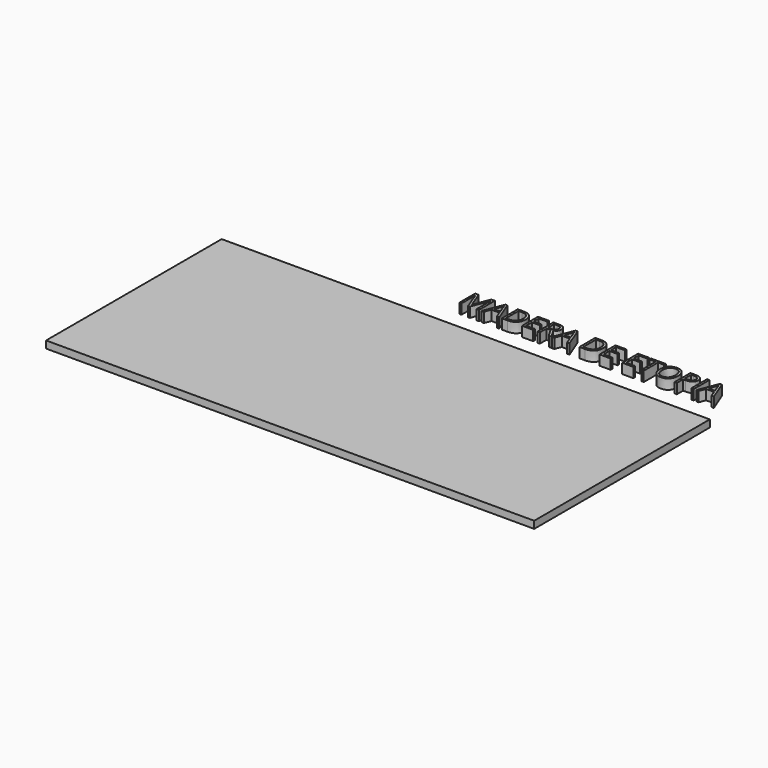
from build123d import *

# Parameters (mm, degrees)
F0_W         = 1223
F0_H         = 550
F1_DEPTH     = 18
F2_TEXT_SIZE = 69.4444444444
F3_DEPTH     = 25


# Not quite as in the source:
# - Text() gives the source's letters only with a copy of the font that has no kerning and outlines rounded to 1/6400 em; it was checked with that copy


with BuildPart() as f1:
    # F0 (on Top) → F1 (new body)
    with BuildSketch(Plane.XY):
        with Locations((611.5, 275)):
            Rectangle(F0_W, F0_H)
    extrude(amount=F1_DEPTH)


with BuildPart() as f3:
    # F2 (on Top) → F3 (new body)
    with BuildSketch(Plane.XY):
        with Locations((532.9559638245, 619.7482676835)):
            Text('MADERA DE ETOPIA', F2_TEXT_SIZE, font='Open Sans', text_align=(TextAlign.LEFT, TextAlign.BOTTOM))
    extrude(amount=F3_DEPTH)


solid = Compound([f1.part, f3.part])
